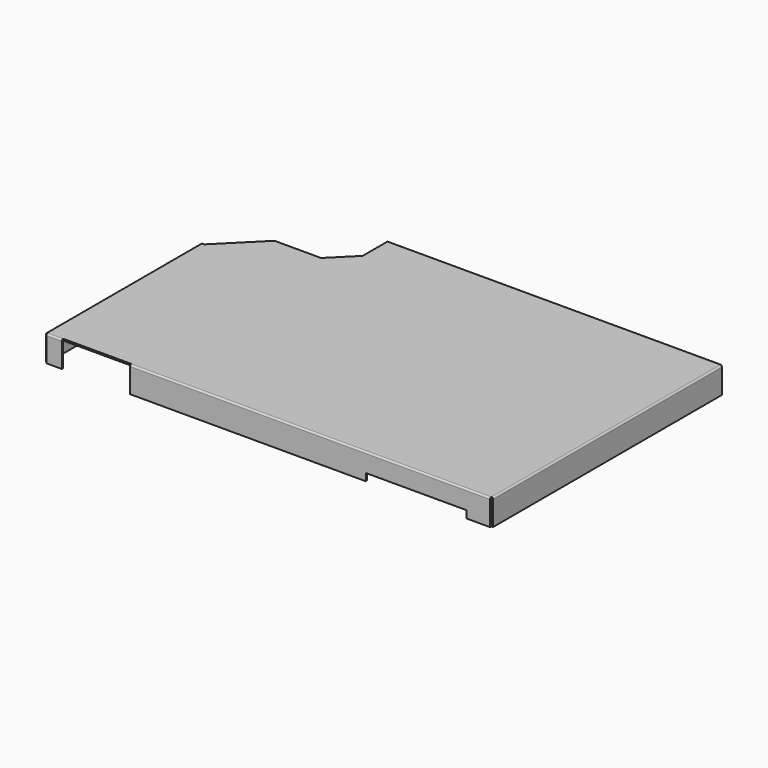
from build123d import *

# Parameters (mm, degrees)
F0_W     = 0.2
F0_H     = 12.3
F0_H_2   = 10
F0_H_3   = 1.5
F1_DEPTH = 3
F0_W_2   = 1.9
F0_H_4   = 0.2
F0_W_3   = 29
F0_W_4   = 2.900001
F0_W_5   = 12.399999
F0_W_6   = 40.999958
F0_H_5   = 35.199967
F2_START = 3
F2_DEPTH = 0.2
F3_DEPTH = 0.9
F4_DEPTH = 0.5
F5_R     = 0.1999


# Not quite as in the source:
# - a fillet or chamfer is up to 0.001 mm smaller than in the source, because OpenCascade refuses the exact size


with BuildPart() as f1:
    # F0 (on Top) → F1 (new body)
    with BuildSketch(Plane.XY):
        with Locations((-26.70002, -11.450007)):
            Rectangle(F0_W, F0_H)
        with Locations((-26.70002, -0.300007)):
            Rectangle(F0_W, F0_H_2)
        with Locations((-26.70002, 5.449993)):
            Rectangle(F0_W, F0_H_3)
    extrude(amount=F1_DEPTH)

    # F0 (on Top) → F4 (cut)
    with BuildSketch(Plane.XY):
        with Locations((-26.70002, -0.300007)):
            Rectangle(F0_W, F0_H_2)
    extrude(amount=F4_DEPTH, mode=Mode.SUBTRACT)


with BuildPart() as f1b:
    # F0 (on Top) → F1, piece 2 (new body)
    with BuildSketch(Plane.XY):
        with Locations((-25.65002, -17.700007)):
            Rectangle(F0_W_2, F0_H_4)
    extrude(amount=F1_DEPTH)


with BuildPart() as f1c:
    # F0 (on Top) → F1, piece 3 (new body)
    with BuildSketch(Plane.XY):
        with Locations((-1.80002, -17.700007)):
            Rectangle(F0_W_3, F0_H_4)
        with Locations((26.5499795, -17.700007)):
            Rectangle(F0_W_4, F0_H_4)
        with Locations((18.8999795, -17.700007)):
            Rectangle(F0_W_5, F0_H_4)
    extrude(amount=F1_DEPTH)

    # F0 (on Top) → F3 (cut)
    with BuildSketch(Plane.XY):
        with Locations((18.8999795, -17.700007)):
            Rectangle(F0_W_5, F0_H_4)
    extrude(amount=F3_DEPTH, mode=Mode.SUBTRACT)


with BuildPart() as f1d:
    # F0 (on Top) → F1, piece 4 (new body)
    with BuildSketch(Plane.XY):
        with Locations((7.500001, 17.69996)):
            Rectangle(F0_W_6, F0_H_4)
    extrude(amount=F1_DEPTH)


with BuildPart() as f1e:
    # F0 (on Top) → F1, piece 5 (new body)
    with BuildSketch(Plane.XY):
        with Locations((28.09998, -2.35e-05)):
            Rectangle(F0_W, F0_H_5)
    extrude(amount=F1_DEPTH)


with BuildPart() as f2:
    # F0 (on Top) → F2 (new body)
    with BuildSketch(Plane.XY.offset(F2_START)):
        with Locations((-26.70002, -11.450007)):
            Rectangle(F0_W, F0_H)
        Polygon((-26.60002, -5.300007), (-26.60002, -17.600007), (-24.70002, -17.600007), (-16.30002, -17.600007), (12.69998, -17.600007), (25.099979, -17.600007), (27.99998, -17.600007), (27.99998, 17.59996), (-12.999978, 17.59996), (-12.999978, 13.84288), (-15.84286, 10.999998), (-21.575756, 10.999998), (-26.375761, 6.199993), (-26.60002, 6.199993), (-26.60002, 4.699993), align=None)
        with Locations((-25.65002, -17.700007)):
            Rectangle(F0_W_2, F0_H_4)
        with Locations((-1.80002, -17.700007)):
            Rectangle(F0_W_3, F0_H_4)
        with Locations((18.8999795, -17.700007)):
            Rectangle(F0_W_5, F0_H_4)
        with Locations((26.5499795, -17.700007)):
            Rectangle(F0_W_4, F0_H_4)
        with Locations((28.09998, -2.35e-05)):
            Rectangle(F0_W, F0_H_5)
        with Locations((7.500001, 17.69996)):
            Rectangle(F0_W_6, F0_H_4)
        with Locations((-26.70002, 5.449993)):
            Rectangle(F0_W, F0_H_3)
        with Locations((-26.70002, -0.300007)):
            Rectangle(F0_W, F0_H_2)
    extrude(amount=F2_DEPTH)

    # F5 (radius 0.2 in the source; OpenCascade refuses exactly that, so slightly less here)
    f5_edges = [f2.edges().sort_by_distance(p)[0] for p in [
        (5.84998, -17.800007, 3.2),
        (-26.80002, -5.700007, 3.2),
        (7.500001, 17.79996, 3.2),
        (28.19998, -2.4e-05, 3.2),
        (-25.65002, -17.800007, 3.2),
    ]]
    fillet(f5_edges, radius=F5_R)


solid = Compound([f1.part, f1b.part, f1c.part, f1d.part, f1e.part, f2.part])
